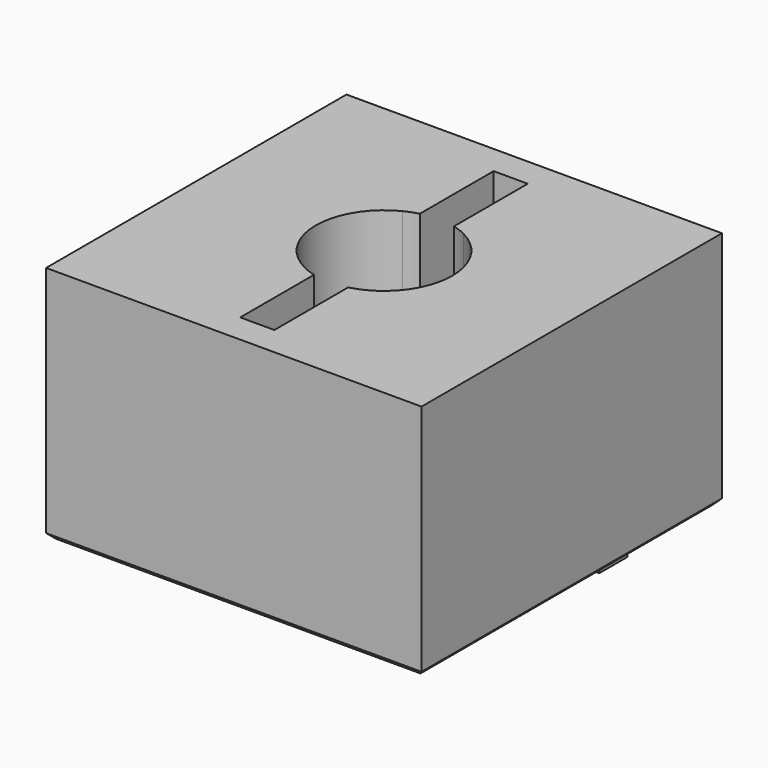
from build123d import *

# Parameters (mm, degrees)
F0_W         = 17.4625
F0_H         = 17.4625
F1_DEPTH     = 11.1125
F3_SIZE      = 0.254
F4_DEPTH     = 9.525
F6_DEPTH     = 0.79375
F5_TEXT_SIZE = 13.0527777778
F7_DEPTH     = 0.79375


# Not quite as in the source:
# - Text() gives the source's letters only with a copy of the font that has no kerning and outlines rounded to 1/6400 em; it was checked with that copy


with BuildPart() as f1:
    # F0 (on Top) → F1 (new body)
    with BuildSketch(Plane.XY):
        Rectangle(F0_W, F0_H)
    extrude(amount=F1_DEPTH)

    # F3
    f3_edges = [f1.edges().sort_by_distance(p)[0] for p in [
        (-8.73125, 0, 0),
        (0, -8.73125, 0),
        (8.73125, 0, 0),
        (0, 8.73125, 0),
    ]]
    chamfer(f3_edges, length=F3_SIZE)

    # F2 (on face) → F4 (cut)
    with BuildSketch(Plane.XY.offset(11.1125)):
        with BuildLine():
            Line((0.79375, 3.0741805311), (0.79375, 7.366))
            Line((0.79375, 7.366), (0, 7.366))
            Line((0, 7.366), (-0.79375, 7.366))
            Line((-0.79375, 7.366), (-0.79375, 3.0741805311))
            ThreePointArc((-0.79375, 3.0741805311), (-1.1135529974, 2.973318806), (-1.4209345682, 2.839290396))
            ThreePointArc((-1.4209345682, 2.839290396), (-3.175, 0), (-1.4209345682, -2.839290396))
            ThreePointArc((-1.4209345682, -2.839290396), (-1.1135529974, -2.973318806), (-0.79375, -3.0741805311))
            Line((-0.79375, -3.0741805311), (-0.79375, -7.366))
            Line((-0.79375, -7.366), (0.79375, -7.366))
            Line((0.79375, -7.366), (0.79375, -3.0741805311))
            ThreePointArc((0.79375, -3.0741805311), (1.1135529974, -2.973318806), (1.4209345682, -2.839290396))
            ThreePointArc((1.4209345682, -2.839290396), (3.175, 0), (1.4209345682, 2.839290396))
            ThreePointArc((1.4209345682, 2.839290396), (1.1135529974, 2.973318806), (0.79375, 3.0741805311))
        make_face()
    extrude(amount=-F4_DEPTH, mode=Mode.SUBTRACT)

    # F5 (on face) → F6 (join)
    with BuildSketch(Plane(origin=(0, 0, 0), x_dir=(1, 0, 0), z_dir=(0, 0, -1))):
        Polygon((1.9164041523, 4.7595882), (1.9164041523, -4.5588714354), (7.6718633537, -4.5588714354), (7.6718633537, -2.9272742132), (3.8926762877, -2.9272742132), (3.8926762877, 4.7595882), align=None)
    extrude(amount=F6_DEPTH)

    # F5 (on face) → F7 (join)
    with BuildSketch(Plane(origin=(0, 0, 0), x_dir=(1, 0, 0), z_dir=(0, 0, -1))):
        with Locations((-7.9629170283, -4.5588714354)):
            Text('XL', F5_TEXT_SIZE, font='Open Sans', font_style=FontStyle.BOLD, text_align=(TextAlign.LEFT, TextAlign.BOTTOM))
    extrude(amount=F7_DEPTH)


solid = f1.part
